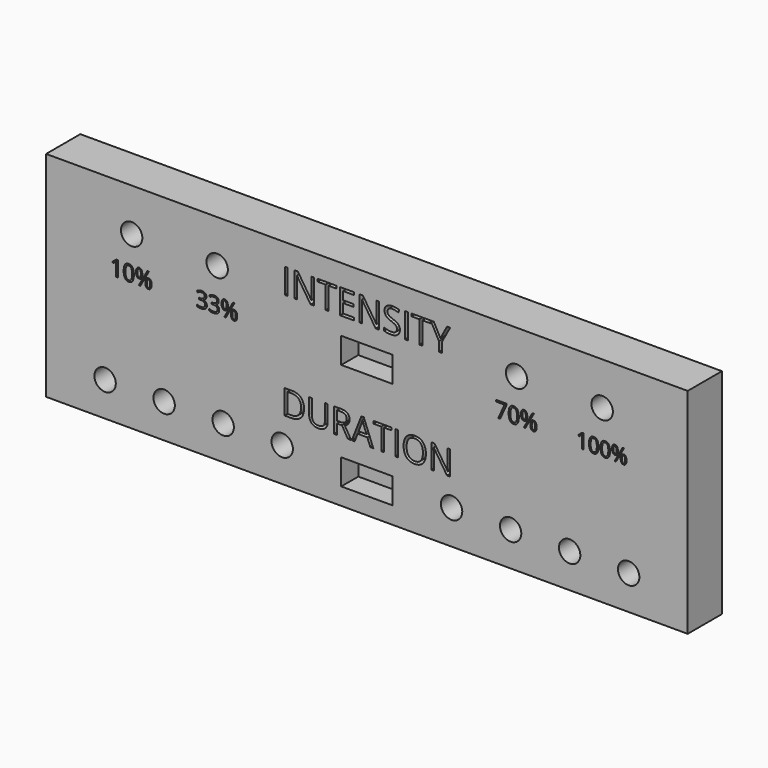
from build123d import *

# Parameters (mm, degrees)
F0_W           = 150
F0_H           = 50
F1_DEPTH       = 10
F2_TEXT_SIZE   = 8.1604029199
F2_TEXT_SIZE_2 = 7.9374922485
F3_DEPTH       = 5
F4_W           = 12
F4_H           = 6
F5_DEPTH       = 5
F6_R           = 2.5
F7_DEPTH       = 5
F8_TEXT_SIZE   = 5.0497080638
F8_TEXT_SIZE_2 = 4.7021367783
F9_DEPTH       = 5
F10_R          = 2.5
F11_DEPTH      = 5


# Not quite as in the source:
# - Text() gives the source's letters only with a copy of the font that has no kerning and outlines rounded to 1/6400 em; it was checked with that copy


with BuildPart() as f1:
    # F0 (on Front) → F1 (new body)
    with BuildSketch(Plane.XZ):
        Rectangle(F0_W, F0_H)
    extrude(amount=F1_DEPTH)

    # F2 (on face) → F3 (cut)
    with BuildSketch(Plane.XZ.offset(10)):
        with Locations((-20, 14.1245098977)):
            Text('INTENSITY', F2_TEXT_SIZE, font='Open Sans', text_align=(TextAlign.LEFT, TextAlign.BOTTOM))
        with Locations((-20, -10.714994419)):
            Text('DURATION', F2_TEXT_SIZE_2, font='Open Sans', text_align=(TextAlign.LEFT, TextAlign.BOTTOM))
    extrude(amount=-F3_DEPTH, mode=Mode.SUBTRACT)

    # F4 (on face) → F5 (cut)
    with BuildSketch(Plane.XZ.offset(10)):
        with Locations((0, 7)):
            Rectangle(F4_W, F4_H)
        with Locations((0, -18)):
            Rectangle(F4_W, F4_H)
    extrude(amount=-F5_DEPTH, mode=Mode.SUBTRACT)

    # F6 (on face) → F7 (cut)
    with BuildSketch(Plane.XZ.offset(10)):
        with Locations((-55, 15)):
            Circle(F6_R)
        with Locations((-35, 15)):
            Circle(F6_R)
        with Locations((35, 15)):
            Circle(F6_R)
        with Locations((55, 15)):
            Circle(F6_R)
    extrude(amount=-F7_DEPTH, mode=Mode.SUBTRACT)

    # F8 (on face) → F9 (cut)
    with BuildSketch(Plane.XZ.offset(10)):
        with Locations((-40, 5)):
            Text('33%', F8_TEXT_SIZE, font='Open Sans', text_align=(TextAlign.LEFT, TextAlign.BOTTOM))
        with Locations((30, 5)):
            Text('70%', F8_TEXT_SIZE, font='Open Sans', text_align=(TextAlign.LEFT, TextAlign.BOTTOM))
        with Locations((49, 5)):
            Text('100%', F8_TEXT_SIZE_2, font='Open Sans', text_align=(TextAlign.LEFT, TextAlign.BOTTOM))
        with Locations((-60, 5)):
            Text('10%', F8_TEXT_SIZE, font='Open Sans', text_align=(TextAlign.LEFT, TextAlign.BOTTOM))
    extrude(amount=-F9_DEPTH, mode=Mode.SUBTRACT)

    # F10 (on face) → F11 (cut)
    with BuildSketch(Plane.XZ.offset(10)):
        with Locations((-61.2, -17)):
            Circle(F10_R)
        with Locations((-47.4, -17)):
            Circle(F10_R)
        with Locations((-33.6, -17)):
            Circle(F10_R)
        with Locations((-19.8, -17)):
            Circle(F10_R)
        with Locations((19.8, -17)):
            Circle(F10_R)
        with Locations((33.6, -17)):
            Circle(F10_R)
        with Locations((47.4, -17)):
            Circle(F10_R)
        with Locations((61.2, -17)):
            Circle(F10_R)
    extrude(amount=-F11_DEPTH, mode=Mode.SUBTRACT)


solid = f1.part
